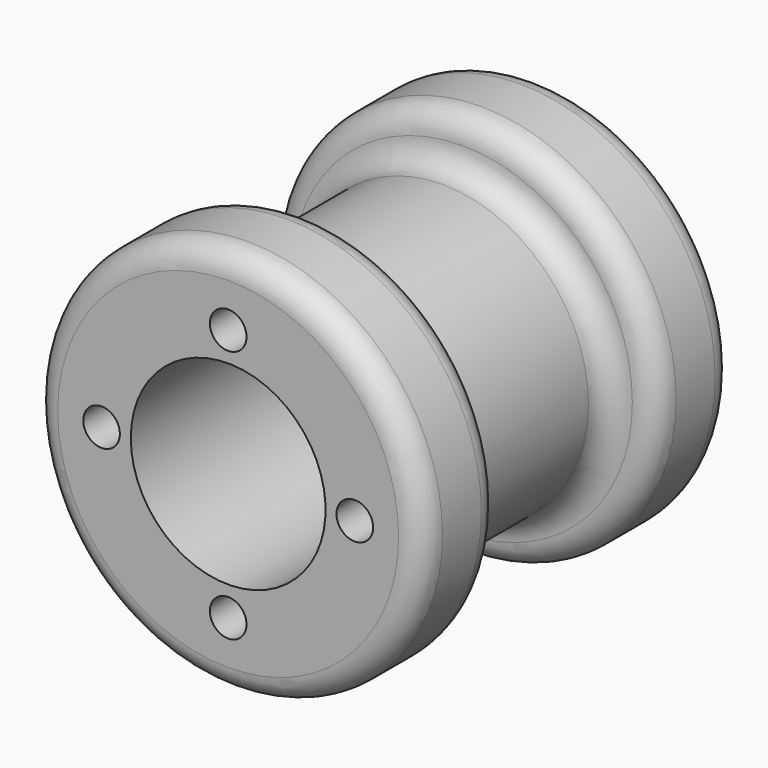
from build123d import *

# Parameters (mm, degrees)
F0_R     = 12.7
F1_DEPTH = 6.35
F2_R     = 9.525
F3_DEPTH = 12.7
F4_R     = 12.7
F5_DEPTH = 6.35
F6_R     = 1.58749
F8_D     = 12.7
F9_D     = 2.3876
F9_DEPTH = 3.175
F9_TIP   = 0.717307407


# Not quite as in the source:
# - a fillet or chamfer is up to 0.001 mm smaller than in the source, because OpenCascade refuses the exact size


with BuildPart() as f1:
    # F0 (on Front) → F1 (new body)
    with BuildSketch(Plane.XZ):
        Circle(F0_R)
    extrude(amount=F1_DEPTH)

    # F2 (on face) → F3 (join)
    with BuildSketch(Plane.XZ.offset(6.35)):
        Circle(F2_R)
    extrude(amount=F3_DEPTH)

    # F4 (on face) → F5 (join)
    with BuildSketch(Plane.XZ.offset(19.05)):
        Circle(F4_R)
    extrude(amount=F5_DEPTH)

    # F6 (radius 1.5875 in the source; OpenCascade refuses exactly that, so slightly less here)
    f6_edges = [f1.edges().sort_by_distance(p)[0] for p in [
        (-12.7, 0, 0),
        (-12.7, -6.35, 0),
        (12.7, -22.225, 0),
        (-12.7, -19.05, 0),
        (-12.7, -25.4, 0),
        (-9.525, -6.35, 0),
        (-9.525, -19.05, 0),
    ]]
    fillet(f6_edges, radius=F6_R)

    # F8 (through all)
    with Locations(Plane.XZ.offset(25.4)):
        with Locations((0, 0)):
            Hole(F8_D / 2)

    # F9
    with Locations(Plane.XZ.offset(25.4)):
        with Locations((0, 8.255), (8.255, 0), (0, -8.255), (-8.255, 0)):
            Hole(F9_D / 2, depth=F9_DEPTH)
            with Locations((0, 0, -(F9_DEPTH + F9_TIP / 2))):  # 118° drill point
                Cone(0, F9_D / 2, F9_TIP, mode=Mode.SUBTRACT)


solid = f1.part
